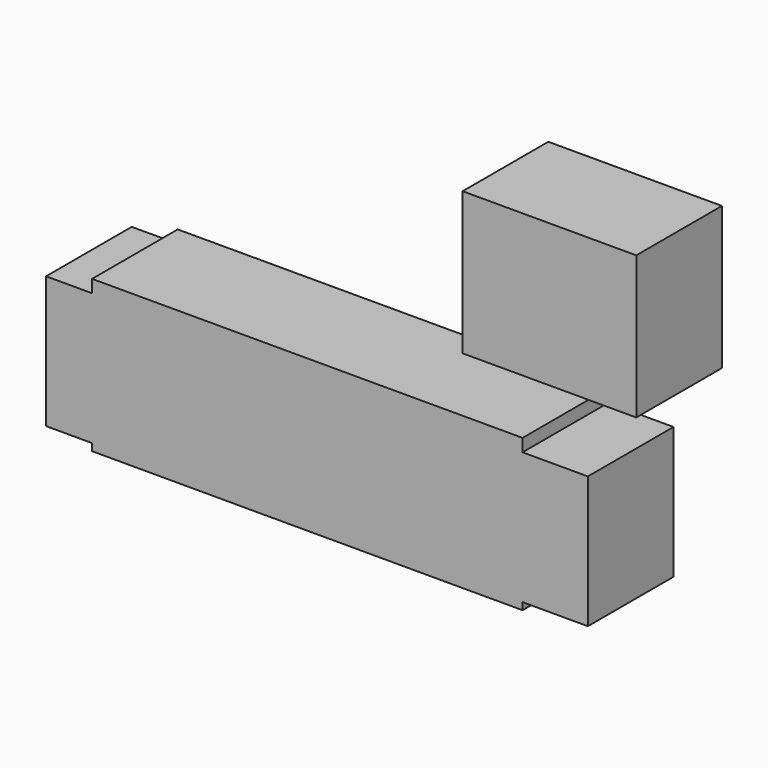
from build123d import *

# Parameters (mm, degrees)
F5_DEPTH = 12.7
F7_DEPTH = 12.7
F2_W     = 128.5309195518
F2_H     = 31.2910405919


# Not quite as in the source:
# - the program builds the solid bodies; features that only make, move or delete a surface that nothing else refers to are left out


with BuildPart() as f5:
    # F3 (on Front) → F5 (new body, symmetric)
    with BuildSketch(Plane.XZ):
        Polygon((35.4110151529, 16.973875463), (-53.555496037, 16.973875463), (-53.555496037, -19.0224424005), (48.5804006457, -19.0224424005), (48.5804006457, 16.973875463), align=None)
    extrude(amount=F5_DEPTH, both=True)

    # F2 (on Front) → F7, piece 2 (join, symmetric)
    with BuildSketch(Plane.XZ):
        with Locations((-0.1980438828, -1.6833790578)):
            Rectangle(F2_W, F2_H)
    extrude(amount=F7_DEPTH, both=True)


with BuildPart() as f7:
    # F2 (on Front) → F7 (new body, symmetric)
    with BuildSketch(Plane.XZ):
        Polygon((34.3607328832, 30.0037506968), (64.0674158931, 30.0037506968), (75.5539983511, 30.0037506968), (75.5539983511, 63.8693645597), (34.3607328832, 63.8693645597), align=None)
    extrude(amount=F7_DEPTH, both=True)


solid = Compound([f5.part, f7.part])
